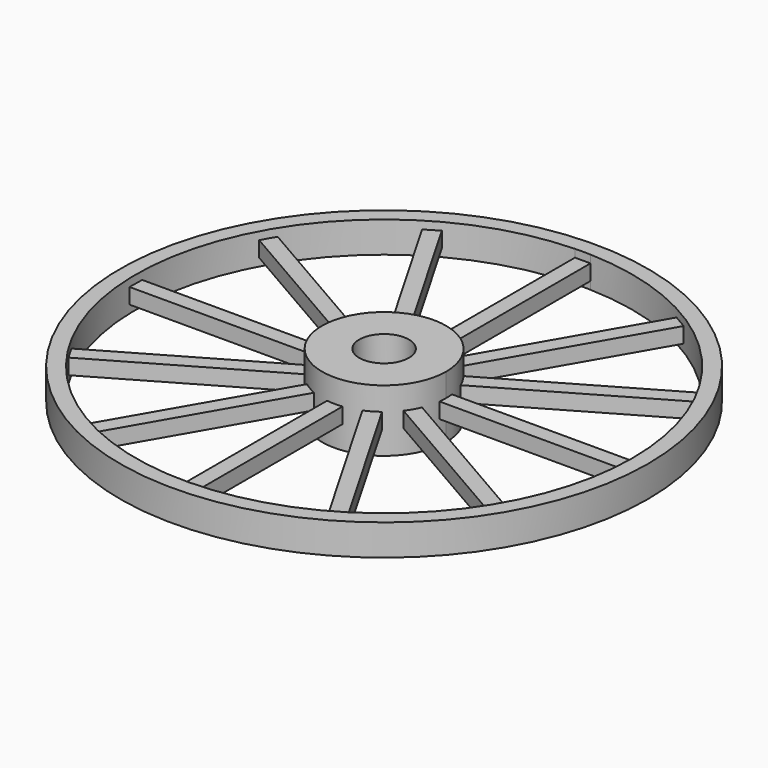
from build123d import *

# Parameters (mm, degrees)
F1_DEPTH      = 10
F2_DEPTH      = 2.5
F3_COUNT      = 12
F3_ANGLE      = 330
F0_R          = 85.039053
F4_DEPTH      = 5
F5_R          = 8
F6_DEPTH      = 10.001
F6_DEPTH_BACK = 25


with BuildPart() as f1:
    # F0 (on Top) → F1 (new body, symmetric)
    with BuildSketch(Plane.XY):
        with BuildLine():
            ThreePointArc((-2.5, 19.843135), (-13.228757, -15), (20, 0))
            ThreePointArc((20, 0), (15, 13.228757), (2.5, 19.843135))
            Line((2.5, 19.843135), (2.5, 0))
            Line((2.5, 0), (-2.5, 0))
            Line((-2.5, 0), (-2.5, 19.843135))
        make_face()
        with BuildLine():
            Line((2.5, 0), (2.5, 19.843135))
            ThreePointArc((2.5, 19.843135), (0, 20), (-2.5, 19.843135))
            Line((-2.5, 19.843135), (-2.5, 0))
            Line((-2.5, 0), (2.5, 0))
        make_face()
    extrude(amount=F1_DEPTH, both=True)

    # F5 (on Top) → F6 (cut, two sides)
    with BuildSketch(Plane.XY) as f6_sk:
        Circle(F5_R)
    extrude(amount=-F6_DEPTH, mode=Mode.SUBTRACT)
    extrude(f6_sk.sketch, amount=F6_DEPTH_BACK, mode=Mode.SUBTRACT)


with BuildPart() as f2:
    # F0 (on Top) → F2 (new body, symmetric)
    with BuildSketch(Plane.XY):
        with BuildLine():
            ThreePointArc((-2.5, 19.843135), (0, 20), (2.5, 19.843135))
            Line((2.5, 19.843135), (2.5, 80))
            Line((2.5, 80), (-2.5, 80))
            Line((-2.5, 80), (-2.5, 19.843135))
        make_face()
    extrude(amount=F2_DEPTH, both=True)


with BuildPart() as f3_1:
    # F3: instance of F2
    add(f2.part.rotate(Axis((0, 0, 10), (0, 0, -1)), 1 * F3_ANGLE / (F3_COUNT - 1)))


with BuildPart() as f3_2:
    # F3: instance of F2
    add(f2.part.rotate(Axis((0, 0, 10), (0, 0, -1)), 2 * F3_ANGLE / (F3_COUNT - 1)))


with BuildPart() as f3_3:
    # F3: instance of F2
    add(f2.part.rotate(Axis((0, 0, 10), (0, 0, -1)), 3 * F3_ANGLE / (F3_COUNT - 1)))


with BuildPart() as f3_4:
    # F3: instance of F2
    add(f2.part.rotate(Axis((0, 0, 10), (0, 0, -1)), 4 * F3_ANGLE / (F3_COUNT - 1)))


with BuildPart() as f3_5:
    # F3: instance of F2
    add(f2.part.rotate(Axis((0, 0, 10), (0, 0, -1)), 5 * F3_ANGLE / (F3_COUNT - 1)))


with BuildPart() as f3_6:
    # F3: instance of F2
    add(f2.part.rotate(Axis((0, 0, 10), (0, 0, -1)), 6 * F3_ANGLE / (F3_COUNT - 1)))


with BuildPart() as f3_7:
    # F3: instance of F2
    add(f2.part.rotate(Axis((0, 0, 10), (0, 0, -1)), 7 * F3_ANGLE / (F3_COUNT - 1)))


with BuildPart() as f3_8:
    # F3: instance of F2
    add(f2.part.rotate(Axis((0, 0, 10), (0, 0, -1)), 8 * F3_ANGLE / (F3_COUNT - 1)))


with BuildPart() as f3_9:
    # F3: instance of F2
    add(f2.part.rotate(Axis((0, 0, 10), (0, 0, -1)), 9 * F3_ANGLE / (F3_COUNT - 1)))


with BuildPart() as f3_10:
    # F3: instance of F2
    add(f2.part.rotate(Axis((0, 0, 10), (0, 0, -1)), 10 * F3_ANGLE / (F3_COUNT - 1)))


with BuildPart() as f3_11:
    # F3: instance of F2
    add(f2.part.rotate(Axis((0, 0, 10), (0, 0, -1)), 11 * F3_ANGLE / (F3_COUNT - 1)))


with BuildPart() as f4:
    # F0 (on Top) → F4 (new body, symmetric)
    with BuildSketch(Plane.XY):
        Circle(F0_R)
        with BuildLine():
            ThreePointArc((-2.5, 80), (0, 80.039053), (2.5, 80))
            ThreePointArc((2.5, 80), (57.473244, 55.705262), (80.039053, 0))
            ThreePointArc((80.039053, 0), (-55.705262, -57.473244), (-2.5, 80))
        make_face(mode=Mode.SUBTRACT)
    extrude(amount=F4_DEPTH, both=True)


solid = Compound([f1.part, f2.part, f3_1.part, f3_2.part, f3_3.part, f3_4.part, f3_5.part, f3_6.part, f3_7.part, f3_8.part, f3_9.part, f3_10.part, f3_11.part, f4.part])
